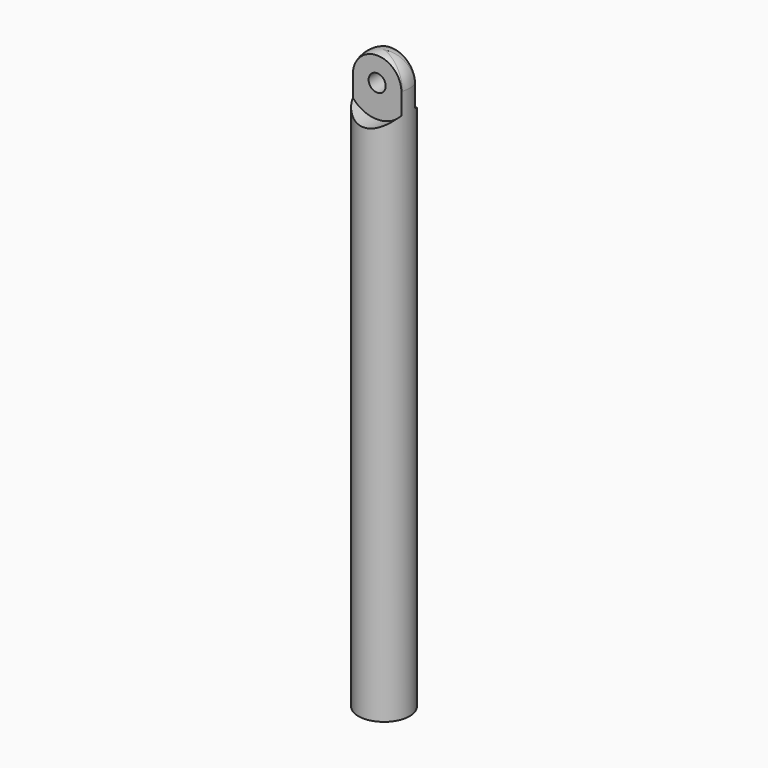
from build123d import *

# Parameters (mm, degrees)
F0_R        = 6
F1_DEPTH    = 135
F3_START    = -2
F3_DEPTH    = 4.0010001005
F4_START    = 2
F4_DEPTH    = 4
F5_T2_ANGLE = 325.4889919963
F5_T4_ANGLE = 306.0016128171
F5_T6_ANGLE = 306.0016128171
F6_R        = 2
F7_DEPTH    = 12.5
F8_R        = 4.8
F9_DEPTH    = 6
F10_R       = 2.375
F11_DEPTH   = 7.5


# Not quite as in the source:
# - a fillet or chamfer that OpenCascade refuses, or shapes differently, is made with other operations: its cross-section is extruded or revolved along the edge and cut away or added


with BuildPart() as f1:
    # F0 (on Top) → F1 (new body)
    with BuildSketch(Plane.XY):
        Circle(F0_R)
    extrude(amount=F1_DEPTH)

    # F2 (on Front) → F3 (cut)
    with BuildSketch(Plane.XZ.offset(F3_START)):
        with BuildLine():
            Line((-6.0225790367, 135.0244730711), (-6.0225790367, 124.5302637944))
            ThreePointArc((-6.0225790367, 124.5302637944), (0.1221735447, 121.5009951577), (6.1649857089, 124.7288232056))
            Line((6.1649857089, 124.7288232056), (6.1649857089, 135.0244730711))
            Line((6.1649857089, 135.0244730711), (-6.0225790367, 135.0244730711))
        make_face()
    extrude(amount=-F3_DEPTH, mode=Mode.SUBTRACT)

    # F2 (on Front) → F4 (cut)
    with BuildSketch(Plane.XZ.offset(F4_START)):
        with BuildLine():
            Line((-6.0225790367, 135.0244730711), (-6.0225790367, 124.5302637944))
            ThreePointArc((-6.0225790367, 124.5302637944), (0.1221735447, 121.5009951577), (6.1649857089, 124.7288232056))
            Line((6.1649857089, 124.7288232056), (6.1649857089, 135.0244730711))
            Line((6.1649857089, 135.0244730711), (-6.0225790367, 135.0244730711))
        make_face()
    extrude(amount=F4_DEPTH, mode=Mode.SUBTRACT)

    # F5: fillet of radius 6 on 3 edges, made by hand

    # F5_s1 → F5_t2 (revolve, cut)
    with BuildSketch(Plane(origin=(0, 0, 0), x_dir=(0, 0, 1), z_dir=(0.2966333156, -0.9549914534, 0))):
        with BuildLine():
            ThreePointArc((128.9990343146, -6.0004), (133.242299252, -4.2429820947), (135.0003999223, 0))
            Line((135.0003999223, 0), (135.6005365042, 0))
            Line((135.6005365042, 0), (135.6001365685, -6))
            Line((135.6001365685, -6), (135, -6.6001365685))
            ThreePointArc((135, -6.6001365685), (131.9995171573, -6.6001365685), (128.9990343146, -6.6005365685))
            Line((128.9990343146, -6.6005365685), (128.9990343146, -6.0004))
        make_face()
    revolve(axis=Axis((0, 0, 135), (0, 0, 1)), revolution_arc=F5_T2_ANGLE, mode=Mode.SUBTRACT)

    # F5_s3 → F5_t4 (revolve, cut)
    with BuildSketch(Plane(origin=(0, 0, 0), x_dir=(0, 0, 1), z_dir=(-0.5981120695, 0.8014124733, 0))):
        with BuildLine():
            ThreePointArc((128.9990343146, -6.0004), (133.242299252, -4.2429820947), (135.0003999223, 0))
            Line((135.0003999223, 0), (135.6005365042, 0))
            Line((135.6005365042, 0), (135.6001365685, -6))
            Line((135.6001365685, -6), (135, -6.6001365685))
            ThreePointArc((135, -6.6001365685), (131.9995171573, -6.6001365685), (128.9990343146, -6.6005365685))
            Line((128.9990343146, -6.6005365685), (128.9990343146, -6.0004))
        make_face()
    revolve(axis=Axis((0, 0, 135), (0, 0, 1)), revolution_arc=F5_T4_ANGLE, mode=Mode.SUBTRACT)

    # F5_s5 → F5_t6 (revolve, cut)
    with BuildSketch(Plane(origin=(0, 0, 0), x_dir=(0, 0, 1), z_dir=(-0.2967679759, 0.9549496157, 0))):
        with BuildLine():
            ThreePointArc((128.9990343146, -6.0004), (133.242299252, -4.2429820947), (135.0003999223, 0))
            Line((135.0003999223, 0), (135.6005365042, 0))
            Line((135.6005365042, 0), (135.6001365685, -6))
            Line((135.6001365685, -6), (135, -6.6001365685))
            ThreePointArc((135, -6.6001365685), (131.9995171573, -6.6001365685), (128.9990343146, -6.6005365685))
            Line((128.9990343146, -6.6005365685), (128.9990343146, -6.0004))
        make_face()
    revolve(axis=Axis((0, 0, 135), (0, 0, 1)), revolution_arc=F5_T6_ANGLE, mode=Mode.SUBTRACT)

    # F6 (on face) → F7 (cut, symmetric)
    with BuildSketch(Plane.XZ):
        with Locations((0, 129)):
            Circle(F6_R)
    extrude(amount=F7_DEPTH, both=True, mode=Mode.SUBTRACT)

    # F8 (on face) → F9 (cut)
    with BuildSketch(Plane(origin=(0, 0, 0), x_dir=(1, 0, 0), z_dir=(0, 0, -1))):
        Circle(F8_R)
    extrude(amount=-F9_DEPTH, mode=Mode.SUBTRACT)

    # F10 (on face) → F11 (join)
    with BuildSketch(Plane(origin=(0, 0, 6), x_dir=(1, 0, 0), z_dir=(0, 0, -1))):
        Circle(F10_R)
    extrude(amount=F11_DEPTH)


solid = f1.part
